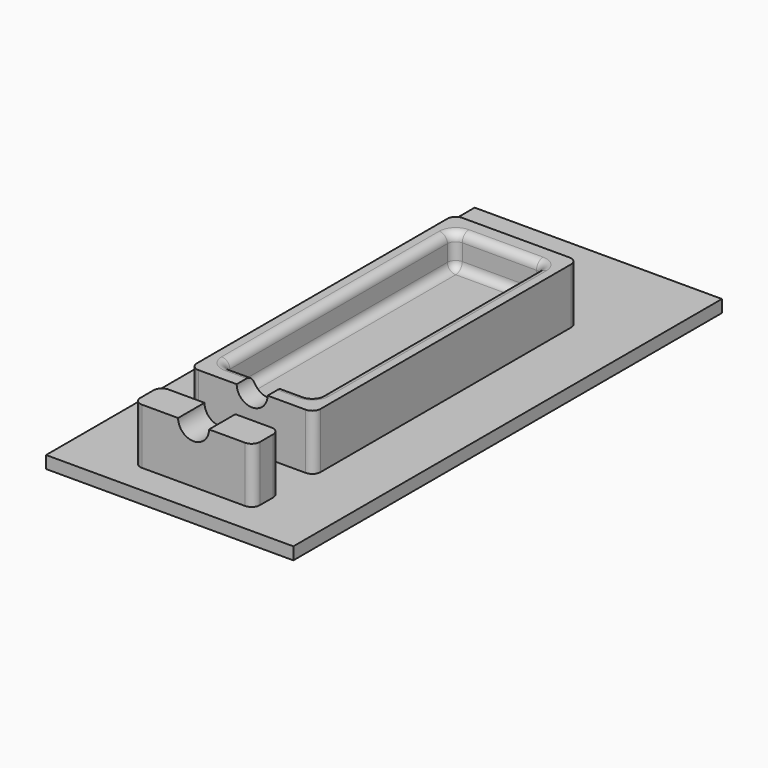
from build123d import *

# Parameters (mm, degrees)
F0_W      = 76.2
F0_H      = 203.2
F1_DEPTH  = 19.05
F2_W      = 55.88
F2_H      = 177.8
F3_DEPTH  = 20.32
F4_F1_R   = 5.08
F4_F2_R   = 5.08
F6_DEPTH  = 25.4
F7_W      = 152.4
F7_H      = 330.2
F7_W_2    = 76.2
F7_H_2    = 203.2
F8_DEPTH  = 3.81
F9_W      = 73.66
F9_H      = 20.32
F10_DEPTH = 34.29
F12_DEPTH = 25.4
F13_R     = 5.08


with BuildPart() as f1:
    # F0 (on Top) → F1 (new body, symmetric)
    with BuildSketch(Plane.XY):
        Rectangle(F0_W, F0_H)
    extrude(amount=F1_DEPTH, both=True)

    # F2 (on face) → F3 (cut)
    with BuildSketch(Plane.XY.offset(19.05)):
        Rectangle(F2_W, F2_H)
    extrude(amount=-F3_DEPTH, mode=Mode.SUBTRACT)

    # F4: fillet of radius 5.08 on 9 edges, made by hand

    # F4_f1
    f4_f1_edges = [f1.edges().sort_by_distance(p)[0] for p in [
        (-27.94, 0, -1.27),
        (0, 88.9, -1.27),
        (27.94, 0, -1.27),
        (0, -88.9, -1.27),
        (-27.94, 88.9, 8.89),
        (27.94, 88.9, 8.89),
        (27.94, -88.9, 8.89),
        (-27.94, -88.9, 8.89),
    ]]
    fillet(f4_f1_edges, radius=F4_F1_R)

    # F4_f2
    f4_f2_edges = [f1.edges().sort_by_distance(p)[0] for p in [
        (0, 88.9, 19.05),
        (26.4521024484, 87.4121024484, 19.05),
        (-26.4521024484, 87.4121024484, 19.05),
    ]]
    fillet(f4_f2_edges, radius=F4_F2_R)

    # F5 (on face) → F6 (cut)
    with BuildSketch(Plane.XZ.offset(101.6)):
        with BuildLine():
            Line((9.525, 19.05), (-9.525, 19.05))
            ThreePointArc((-9.525, 19.05), (0, 9.525), (9.525, 19.05))
        make_face()
    extrude(amount=-F6_DEPTH, mode=Mode.SUBTRACT)

    # F7 (on face) → F8 (join, symmetric)
    with BuildSketch(Plane(origin=(0, 0, -19.05), x_dir=(1, 0, 0), z_dir=(0, 0, -1))):
        Rectangle(F7_W, F7_H)
        Rectangle(F7_W_2, F7_H_2, mode=Mode.SUBTRACT)
        Rectangle(F7_W_2, F7_H_2)
    extrude(amount=F8_DEPTH, both=True)

    # F9 (on face) → F10 (join)
    with BuildSketch(Plane.XY.offset(-15.24)):
        with Locations((0, -136.5740124)):
            Rectangle(F9_W, F9_H)
    extrude(amount=F10_DEPTH)

    # F11 (on face) → F12 (cut)
    with BuildSketch(Plane.XZ.offset(146.7340124)):
        with BuildLine():
            Line((9.525, 19.05), (-9.525, 19.05))
            ThreePointArc((-9.525, 19.05), (0, 9.525), (9.525, 19.05))
        make_face()
    extrude(amount=-F12_DEPTH, mode=Mode.SUBTRACT)

    # F13
    f13_edges = [f1.edges().sort_by_distance(p)[0] for p in [
        (38.1, -101.6, 1.905),
        (36.83, -126.414012, 1.905),
        (36.83, -146.734012, 1.905),
        (-36.83, -146.734012, 1.905),
        (-36.83, -126.414012, 1.905),
        (-38.1, -101.6, 1.905),
        (38.1, 101.6, 1.905),
        (-38.1, 101.6, 1.905),
    ]]
    fillet(f13_edges, radius=F13_R)


solid = f1.part
